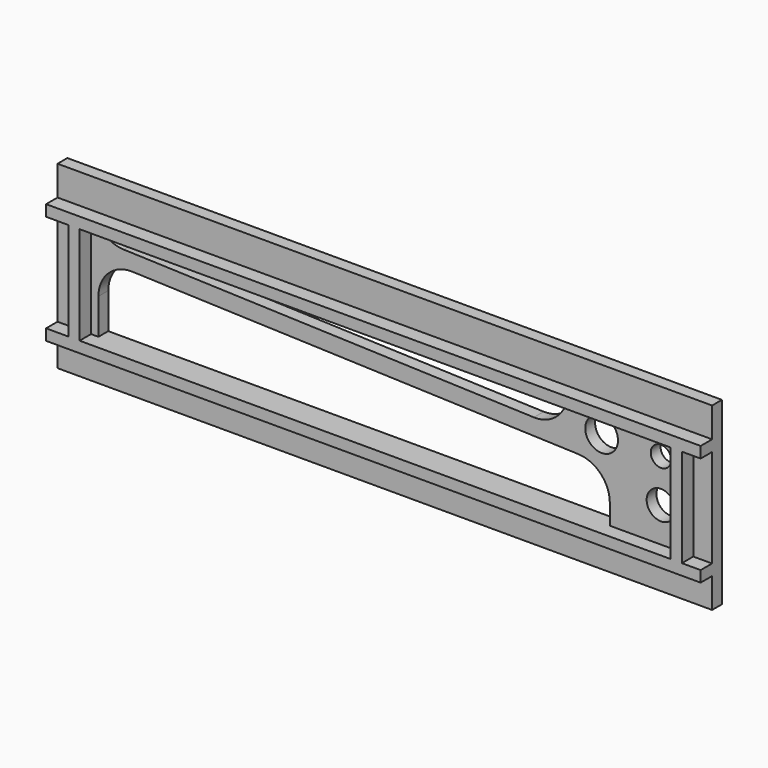
from build123d import *

# Parameters (mm, degrees)
F0_R        = 2.2225
F0_R_2      = 2.54
F0_R_3      = 1.5875
F0_W        = 79.375
F0_H        = 6.35
F1_DEPTH    = 0.9525
F2_T1_DEPTH = 1.905
F3_W        = 3.4798
F3_H        = 1.7145
F3_W_2      = 1.7272
F3_H_2      = 15.24
F3_W_3      = 91.7488066308
F3_H_3      = 1.7272
F3_W_4      = 2.9169933692
F4_DEPTH    = 3.175


# Not quite as in the source:
# - a fillet or chamfer that OpenCascade refuses, or shapes differently, is made with other operations: its cross-section is extruded or revolved along the edge and cut away or added
# - a feature names something its author has since deleted; it is built from what else it names


with BuildPart() as f1:
    # F0 (on Front) → F1 (new body, symmetric)
    with BuildSketch(Plane.XZ):
        Polygon((-50.8, 27.94), (-50.8, 0), (-44.45, 0), (-44.45, 6.35), (-44.45, 17.145), (34.925, 14.3731639216), (34.925, 6.35), (34.925, 0), (50.8, 0), (50.8, 27.94), align=None)
        with Locations((42.8625, 11.7475)):
            Circle(F0_R, mode=Mode.SUBTRACT)
        Polygon((-44.45, 21.59), (28.3304192035, 21.59), (28.3304192035, 17.145), (-44.45, 19.6865482425), align=None, mode=Mode.SUBTRACT)
        with Locations((33.655, 18.415)):
            Circle(F0_R_2, mode=Mode.SUBTRACT)
        with Locations((42.8625, 18.415)):
            Circle(F0_R_3, mode=Mode.SUBTRACT)
        with Locations((-4.7625, 3.175)):
            Rectangle(F0_W, F0_H)
    extrude(amount=F1_DEPTH, both=True)

    # F2: fillet of radius 5.08 on 4 edges, made by hand

    # F2_s2 → F2_t1 (join)
    with BuildSketch(Plane.XZ.offset(-0.9525)):
        with BuildLine():
            ThreePointArc((-39.1927105568, 16.9614114072), (-42.8988645219, 15.5387521917), (-44.45, 11.8845060059))
            Line((-44.45, 11.8845060059), (-44.45, 17.145))
            Line((-44.45, 17.145), (-39.1927105568, 16.9614114072))
        make_face()
        with BuildLine():
            ThreePointArc((34.925, 9.4674649456), (33.4992461857, 12.9963294675), (30.0222894432, 14.5443703468))
            Line((30.0222894432, 14.5443703468), (34.925, 14.3731639216))
            Line((34.925, 14.3731639216), (34.925, 9.4674649456))
        make_face()
        with BuildLine():
            ThreePointArc((-44.45, 21.59), (-42.7347440797, 20.1271540197), (-40.5553991831, 19.5505457851))
            Line((-40.5553991831, 19.5505457851), (-44.45, 19.6865482425))
            Line((-44.45, 19.6865482425), (-44.45, 21.59))
        make_face()
        with BuildLine():
            ThreePointArc((28.3304192035, 21.59), (26.5399663684, 18.4773950775), (23.1386411982, 17.326300883))
            Line((23.1386411982, 17.326300883), (28.3304192035, 17.145))
            Line((28.3304192035, 17.145), (28.3304192035, 21.59))
        make_face()
    extrude(amount=F2_T1_DEPTH)

    # F3 (on Front) → F4 (join)
    with BuildSketch(Plane.XZ):
        with Locations((-49.0601, 5.49275)):
            Rectangle(F3_W, F3_H)
        with Locations((-46.4566, 13.97)):
            Rectangle(F3_W_2, F3_H_2)
        with Locations((-46.4566, 5.49275)):
            Rectangle(F3_W_2, F3_H)
        with Locations((0.2814033154, 5.49275)):
            Rectangle(F3_W_3, F3_H)
        with Locations((-46.4566, 22.4536)):
            Rectangle(F3_W_2, F3_H_3)
        with Locations((-49.0601, 22.4536)):
            Rectangle(F3_W, F3_H_3)
        with Locations((47.0194066308, 13.97)):
            Rectangle(F3_W_2, F3_H_2)
        with Locations((47.0194066308, 5.49275)):
            Rectangle(F3_W_2, F3_H)
        with Locations((0.2814033154, 22.4536)):
            Rectangle(F3_W_3, F3_H_3)
        with Locations((49.3415033154, 5.49275)):
            Rectangle(F3_W_4, F3_H)
        with Locations((47.0194066308, 22.4536)):
            Rectangle(F3_W_2, F3_H_3)
        with Locations((49.3415033154, 22.4536)):
            Rectangle(F3_W_4, F3_H_3)
    extrude(amount=F4_DEPTH)


solid = f1.part
